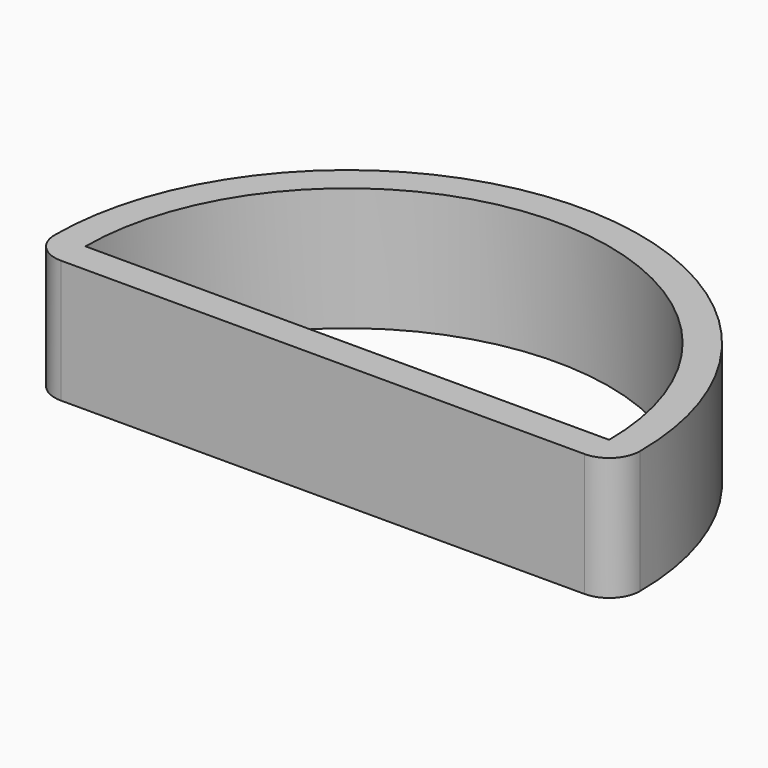
from build123d import *

# Parameters (mm, degrees)
F1_DEPTH = 2
F2_R     = 0.5


with BuildPart() as f1:
    # F0 (on Top) → F1 (new body)
    with BuildSketch(Plane.XY):
        with BuildLine():
            ThreePointArc((-42.5555160352, 38.8332652748), (-47.2791269422, 44.0832652748), (-52.0027378491, 38.8332652748))
            Line((-52.0027378491, 38.8332652748), (-42.5555160352, 38.8332652748))
        make_face()
        with BuildLine():
            ThreePointArc((-51.5291269422, 39.3332652748), (-47.2791269422, 43.5832652748), (-43.0291269422, 39.3332652748))
            Line((-43.0291269422, 39.3332652748), (-51.5291269422, 39.3332652748))
        make_face(mode=Mode.SUBTRACT)
    extrude(amount=F1_DEPTH)

    # F2
    f2_edges = [f1.edges().sort_by_distance(p)[0] for p in [
        (-52.002738, 38.833265, 1),
        (-42.555516, 38.833265, 1),
    ]]
    fillet(f2_edges, radius=F2_R)


solid = f1.part
